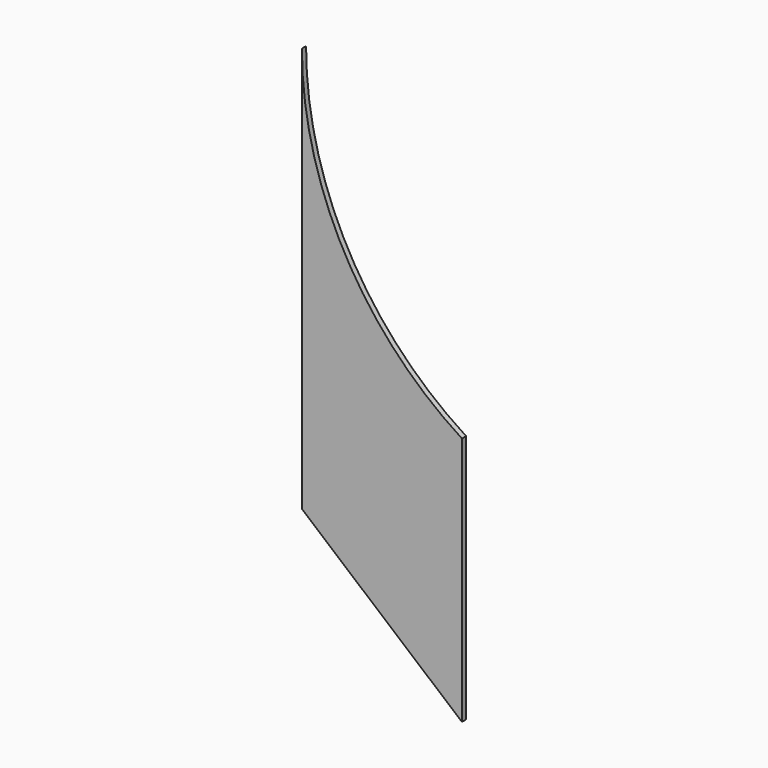
from build123d import *

# Parameters (mm, degrees)
F1_DEPTH = 1.5875


# Not quite as in the source:
# - a length typed as a fraction of an inch, garbled in the dataset ("3 / 203.2 mm" for 3/8 in), is restored


with BuildPart() as f1:
    # F0 (on Front) → F1 (new body)
    with BuildSketch(Plane.XZ):
        with BuildLine():
            ThreePointArc((48.8543696702, -31.1556309462), (13.0177004808, 7.0429102473), (0, 57.7768720686))
            Line((0, 57.7768720686), (0, -65.968029201))
            Line((0, -65.968029201), (48.8543696702, -65.968029201))
            Line((48.8543696702, -65.968029201), (48.8543696702, -31.1556309462))
        make_face()
        Polygon((48.8543696702, -65.968029201), (0, -65.968029201), (48.8543696702, -107.3181778193), align=None)
    extrude(amount=F1_DEPTH)


solid = f1.part
